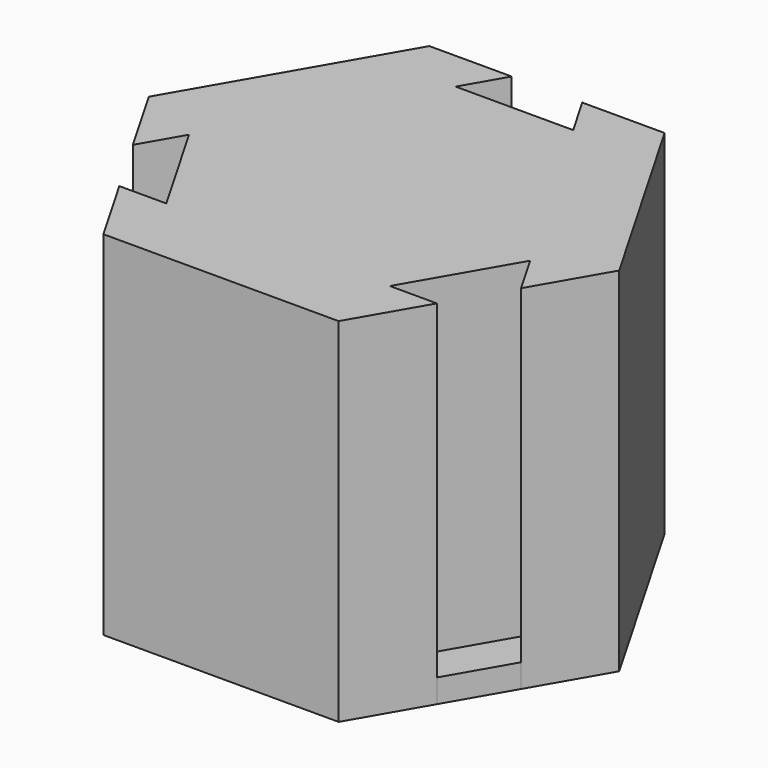
from build123d import *

# Parameters (mm, degrees)
F0_R     = 1.75
F1_DEPTH = 30
F2_DEPTH = 2
F3_START = 28
F3_DEPTH = 2


# Not quite as in the source:
# - ends of sketch curves that miss each other by under 0.0002 mm in the source are joined


with BuildPart() as f1:
    # F0 (on Top) → F1 (new body)
    with BuildSketch(Plane.XY):
        Polygon((-10, -17.3205080757), (10, -17.3205080757), (13.500000035, -11.2583301886), (9.5000001398, -11.2583302492), (14.5000001398, -2.5980762114), (16.5000001398, -6.0621778265), (20, 0), (10, 17.3205080757), (3, 17.3205080757), (5, 13.8564064606), (-5, 13.8564064606), (-3, 17.3205080757), (-10, 17.3205080757), (-20, 0), (-16.4999999301, -6.0621779476), (-14.4999999301, -2.5980763325), (-9.4999999301, -11.2583303703), (-13.4999999301, -11.2583303703), align=None)
        Circle(F0_R, mode=Mode.SUBTRACT)
    extrude(amount=F1_DEPTH)

    # F0 (on Top) → F2 (join)
    with BuildSketch(Plane.XY):
        Polygon((-16.4999999301, -6.0621779476), (-13.4999999301, -11.2583303703), (-9.4999999301, -11.2583303703), (-14.4999999301, -2.5980763325), align=None)
        Polygon((5, 13.8564064606), (3, 17.3205080757), (-3, 17.3205080757), (-5, 13.8564064606), align=None)
        Polygon((9.5000001398, -11.2583302492), (13.5000001398, -11.2583302492), (16.500000035, -6.0621777659), (14.5000001398, -2.5980762114), align=None)
    extrude(amount=F2_DEPTH)

    # F0 (on Top) → F3 (join)
    with BuildSketch(Plane.XY.offset(F3_START)):
        Circle(F0_R)
    extrude(amount=F3_DEPTH)


solid = f1.part
